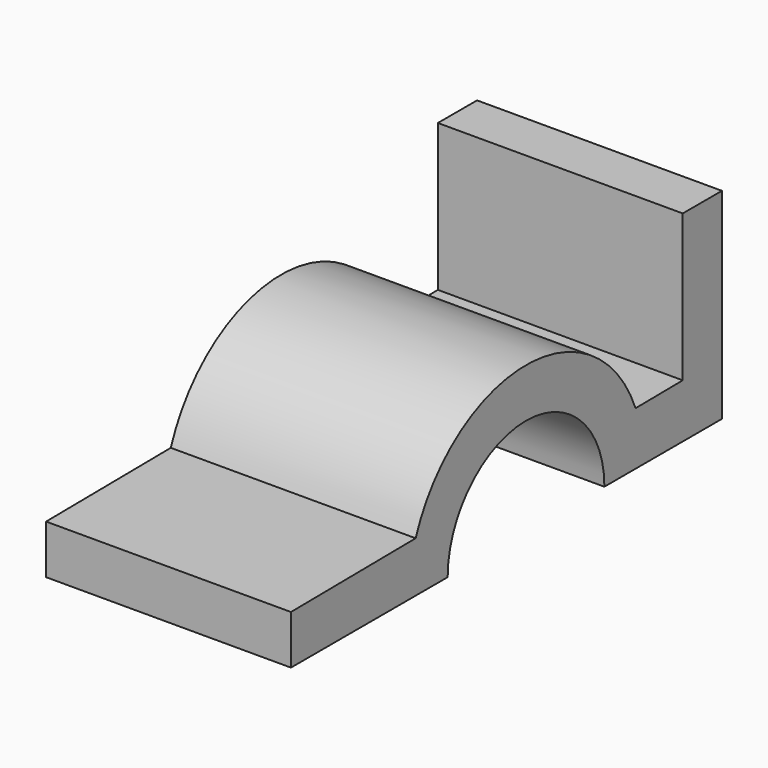
from build123d import *

# Parameters (mm, degrees)
F1_DEPTH = 50


# Not quite as in the source:
# - a feature names something its author has since deleted; it is built from what else it names


with BuildPart() as f1:
    # F0 (on Right) → F1 (new body)
    with BuildSketch(Plane.YZ):
        with BuildLine():
            Line((20.0000005408, 0), (50, 0))
            Line((50, 0), (50, 41))
            Line((50, 41), (40, 41))
            Line((40, 41), (40, 11))
            Line((40, 11), (27.9577328728, 10.8795773287))
            ThreePointArc((27.9577328728, 10.8795773287), (-0.2999844603, 29.9985001125), (-28.1697105934, 10.3183028941))
            Line((-28.1697105934, 10.3183028941), (-60, 10))
            Line((-60, 10), (-60, 0))
            Line((-60, 0), (-19.9999994592, 0))
            ThreePointArc((-19.9999994592, 0), (5.408e-07, 20), (20.0000005408, 0))
        make_face()
    extrude(amount=F1_DEPTH)


solid = f1.part
